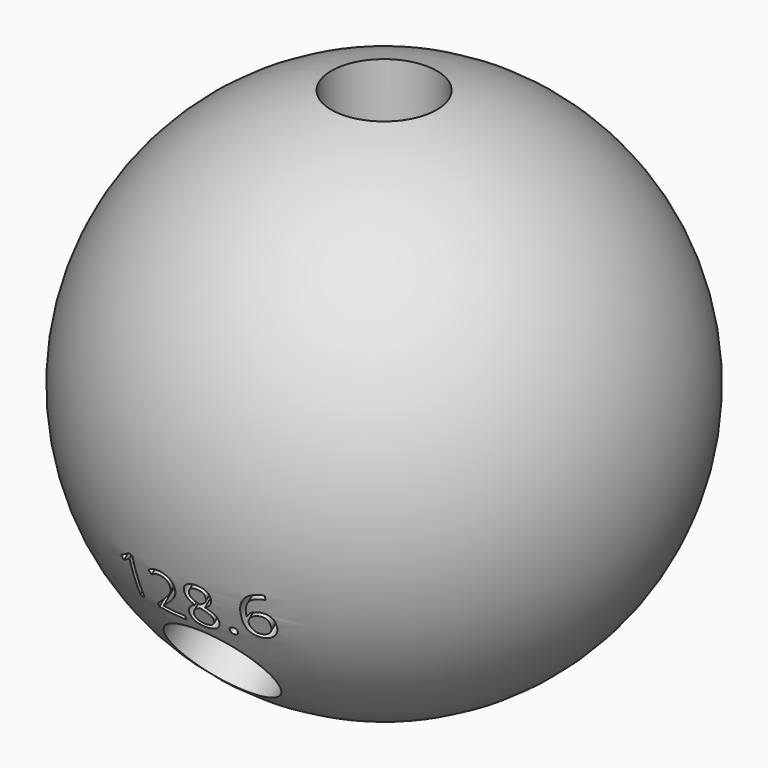
from build123d import *

# Parameters (mm, degrees)
F4_R          = 3.175
F5_DEPTH      = 50.8
F7_ANGLE      = 128.6
F8_ANGLE      = -118.8
F10_TEXT_SIZE = 3.6769132647
F11_DEPTH     = 19.05
F13_TEXT_SIZE = 3.278460483
F14_DEPTH     = 19.05


# Not quite as in the source:
# - Text() gives the source's letters only with a copy of the font that has no kerning and outlines rounded to 1/6400 em; it was checked with that copy


with BuildPart() as f2:
    # F0 (on Front) → F2 (revolve)
    with BuildSketch(Plane.XZ):
        with BuildLine():
            Line((0, -15.875), (0, 15.875))
            ThreePointArc((0, 15.875), (-15.875, 0), (0, -15.875))
        make_face()
    revolve(axis=Axis((0, 0, 0), (0, 0, 1)))

    # F10 (on offset) → F11 (cut)
    with BuildSketch(Plane(origin=(0, -19.8506199994, -15.8465417564), x_dir=(1, 0, 0), z_dir=(0, -0.7815204724, -0.6238795967))):
        with Locations((-4.4026998803, 3.6502513103)):
            Text('128.6', F10_TEXT_SIZE, font='Open Sans', text_align=(TextAlign.LEFT, TextAlign.BOTTOM))
    extrude(amount=-F11_DEPTH, mode=Mode.SUBTRACT)

    # F13 (on offset) → F14 (cut)
    with BuildSketch(Plane(origin=(0, 22.2581896731, -12.2365433222), x_dir=(-1, 0, 0), z_dir=(0, 0.87630668, -0.4817536741))):
        with Locations((-4.235918168, 3.5686311312)):
            Text('118.8', F13_TEXT_SIZE, font='Open Sans', text_align=(TextAlign.LEFT, TextAlign.BOTTOM))
    extrude(amount=-F14_DEPTH, mode=Mode.SUBTRACT)


with BuildPart() as f5:
    # F4 (on offset) → F5 (new body)
    with BuildSketch(Plane.XY.offset(6.35)):
        Circle(F4_R)
    extrude(amount=F5_DEPTH)


with BuildPart() as f7_1:
    # F7: copy of F5
    add(f5.part.rotate(Axis((26.915807277, 0, 0), (1, 0, 0)), F7_ANGLE))


with BuildPart() as f8_1:
    # F8: copy of F5
    add(f5.part.rotate(Axis((26.915807277, 0, 0), (1, 0, 0)), F8_ANGLE))


with BuildPart() as f2_1:
    add(f2.part)

    # F15: cut F5, F7_1, F8_1
    add(f5.part, mode=Mode.SUBTRACT)
    add(f7_1.part, mode=Mode.SUBTRACT)
    add(f8_1.part, mode=Mode.SUBTRACT)


solid = f2_1.part
